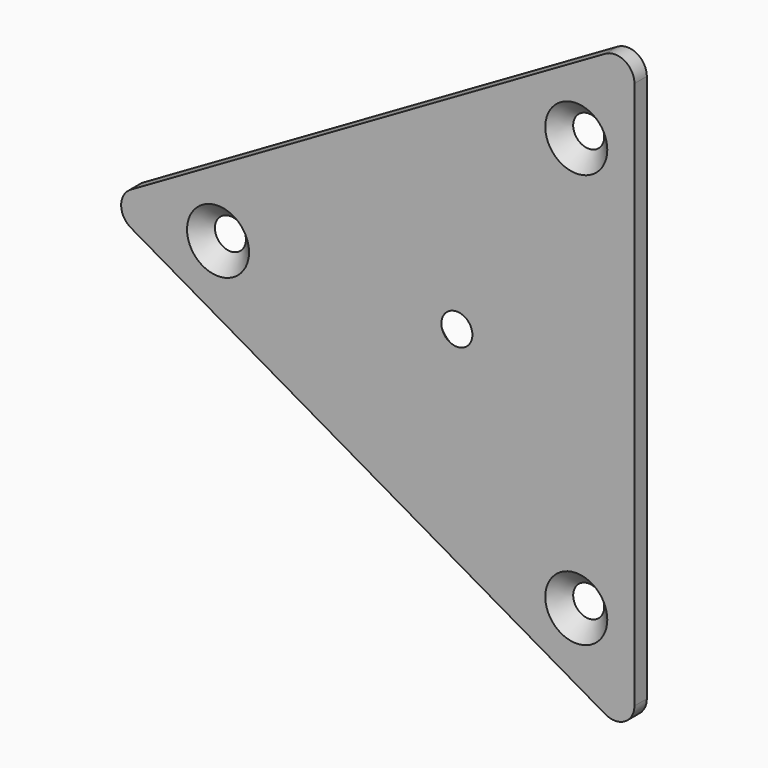
from build123d import *

# Parameters (mm, degrees)
F0_R     = 3
F1_DEPTH = 4
F2_R     = 5


# Not quite as in the source:
# - a fillet or chamfer that OpenCascade refuses, or shapes differently, is made with other operations: its cross-section is extruded or revolved along the edge and cut away or added


with BuildPart() as f1:
    # F0 (on Front) → F1 (new body)
    with BuildSketch(Plane.XZ):
        Polygon((45.8173750394, -79.3580214376), (45.8173750394, 79.3580214376), (-91.6347500787, 0), align=None)
        with Locations((30.8173750394, -53.3772593241)):
            Circle(F0_R, mode=Mode.SUBTRACT)
        with Locations((-61.6347500787, 0)):
            Circle(F0_R, mode=Mode.SUBTRACT)
        Circle(F0_R, mode=Mode.SUBTRACT)
        with Locations((30.8173750394, 53.3772593241)):
            Circle(F0_R, mode=Mode.SUBTRACT)
    extrude(amount=F1_DEPTH)

    # F2
    f2_edges = [f1.edges().sort_by_distance(p)[0] for p in [
        (45.817375, -2, 79.358021),
        (45.817375, -2, -79.358021),
        (-91.63475, -2, 0),
    ]]
    fillet(f2_edges, radius=F2_R)

    # F3: chamfer of 5 on 4 edges, made by hand

    # F3_s1 → F3_t2 (revolve, cut)
    with BuildSketch(Plane.XY):
        Polygon((8, 0), (3, -5), (3, 0), align=None)
    revolve(axis=Axis((0, 0, 0), (0, -1, 0)), mode=Mode.SUBTRACT)

    # F3_s3 → F3_t4 (revolve, cut)
    with BuildSketch(Plane.XY):
        Polygon((-53.6347500787, -4), (-58.6347500787, 1), (-58.6347500787, -4), align=None)
    revolve(axis=Axis((-61.6347500787, -4, 0), (0, -1, 0)), mode=Mode.SUBTRACT)

    # F3_s5 → F3_t6 (revolve, cut)
    with BuildSketch(Plane.XY.offset(53.3772593241)):
        Polygon((38.8173750394, -4), (33.8173750394, 1), (33.8173750394, -4), align=None)
    revolve(axis=Axis((30.8173750394, -4, 53.3772593241), (0, -1, 0)), mode=Mode.SUBTRACT)

    # F3_s7 → F3_t8 (revolve, cut)
    with BuildSketch(Plane.XY.offset(-53.3772593241)):
        Polygon((38.8173750394, -4), (33.8173750394, 1), (33.8173750394, -4), align=None)
    revolve(axis=Axis((30.8173750394, -4, -53.3772593241), (0, -1, 0)), mode=Mode.SUBTRACT)


solid = f1.part
